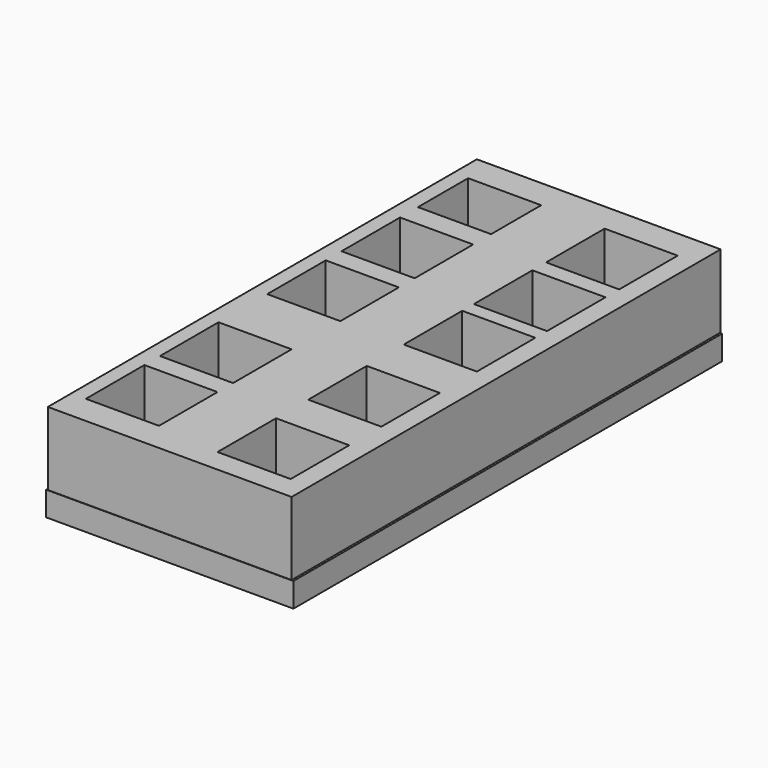
from build123d import *

# Parameters (mm, degrees)
F0_W     = 27.94
F0_H     = 139.7
F0_W_2   = 19.05
F0_H_2   = 19.05
F0_H_3   = 16.3293534029
F0_W_3   = 7.62
F1_DEPTH = 25.4
F2_W     = 64.4415542483
F2_H     = 139.5248323679
F3_DEPTH = 6.35


with BuildPart() as f1:
    # F0 (on Top) → F1 (new body)
    with BuildSketch(Plane.XY):
        with Locations((-17.78, 0)):
            Rectangle(F0_W, F0_H)
        with Locations((-18.415, -52.705)):
            Rectangle(F0_W_2, F0_H_2, mode=Mode.SUBTRACT)
        with Locations((-18.415, -28.575)):
            Rectangle(F0_W_2, F0_H_2, mode=Mode.SUBTRACT)
        with Locations((-18.415, 6.35)):
            Rectangle(F0_W_2, F0_H_2, mode=Mode.SUBTRACT)
        with Locations((-18.415, 30.5456899792)):
            Rectangle(F0_W_2, F0_H_2, mode=Mode.SUBTRACT)
        with Locations((-18.415, 54.0653232986)):
            Rectangle(F0_W_2, F0_H_3, mode=Mode.SUBTRACT)
        Rectangle(F0_W_3, F0_H)
        with Locations((17.78, 0)):
            Rectangle(F0_W, F0_H)
        with Locations((17.145, -54.2791421771)):
            Rectangle(F0_W_2, F0_H_2, mode=Mode.SUBTRACT)
        with Locations((17.145, -24.7503119767)):
            Rectangle(F0_W_2, F0_H_2, mode=Mode.SUBTRACT)
        with Locations((17.145, 6.35)):
            Rectangle(F0_W_2, F0_H_2, mode=Mode.SUBTRACT)
        with Locations((17.145, 29.1921038866)):
            Rectangle(F0_W_2, F0_H_2, mode=Mode.SUBTRACT)
        with Locations((17.145, 52.705)):
            Rectangle(F0_W_2, F0_H_2, mode=Mode.SUBTRACT)
    extrude(amount=F1_DEPTH)

    # F2 (on Top) → F3 (join)
    with BuildSketch(Plane.XY):
        with Locations((0.0985339284, -0.1970678568)):
            Rectangle(F2_W, F2_H)
    extrude(amount=F3_DEPTH)


solid = f1.part
